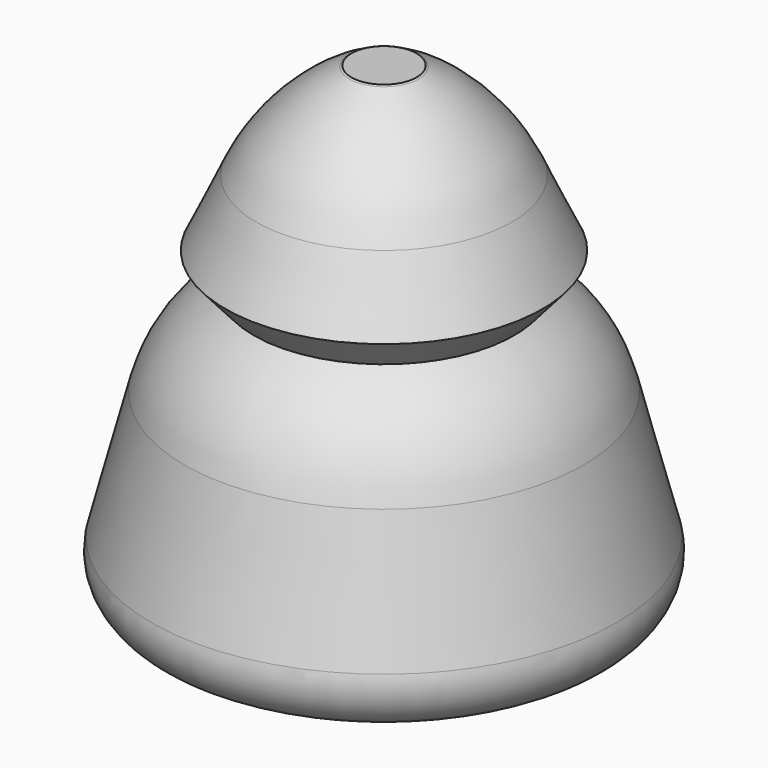
from build123d import *

# Parameters (mm, degrees)
F3_R = 6.8209108122
F4_R = 1.6096783158


# Not quite as in the source:
# - a fillet or chamfer that OpenCascade refuses, or shapes differently, is made with other operations: its cross-section is extruded or revolved along the edge and cut away or added


with BuildPart() as f1:
    # F0 (on Front) → F1 (revolve)
    with BuildSketch(Plane.XZ):
        Polygon((-8.3269113675, 0), (0, 0), (0, 15.9264262766), (-1.0918058688, 15.9264262766), (-3.2759886235, 14.8343360052), (-5.3236596286, 10.4659702629), (-4.3680798262, 9.3738790601), (-6.006217096, 8.9643457904), align=None)
    revolve(axis=Axis((0, 0, 7.9632131383), (0, 0, -1)))

    # F2: fillet of radius 5 on 1 edges, made by hand

    # F2_s1 → F2_t2 (revolve, cut)
    with BuildSketch(Plane.XZ):
        with BuildLine():
            ThreePointArc((-4.3680798262, 9.3738790601), (-5.8387408469, 8.0723577213), (-6.6947110993, 6.3048406604))
            Line((-6.6947110993, 6.3048406604), (-6.006217096, 8.9643457904))
            Line((-6.006217096, 8.9643457904), (-4.3680798262, 9.3738790601))
        make_face()
    revolve(axis=Axis((0, 0, 8.9643457904), (0, 0, -1)), mode=Mode.SUBTRACT)

    # F3
    f3_edges = [f1.edges().sort_by_distance(p)[0] for p in [
        (3.275989, 0, 14.834336),
    ]]
    fillet(f3_edges, radius=F3_R)

    # F4
    f4_edges = [f1.edges().sort_by_distance(p)[0] for p in [
        (8.326911, 0, 0),
    ]]
    fillet(f4_edges, radius=F4_R)


solid = f1.part
